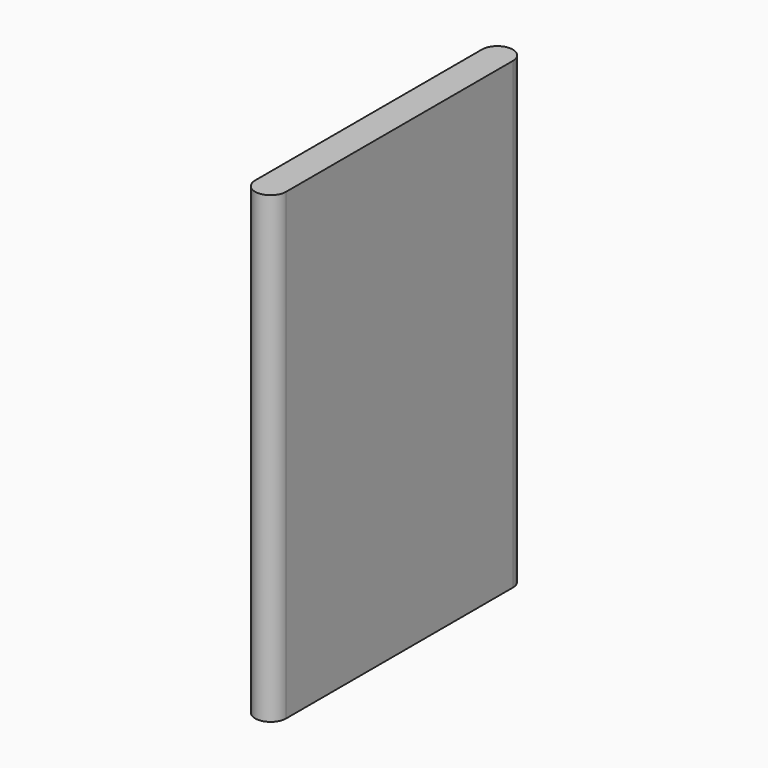
from build123d import *

# Parameters (mm, degrees)
F1_DEPTH     = 90
F2_TEXT_SIZE = 16.9558881971
F3_DEPTH     = 0.5


# Not quite as in the source:
# - Text() gives the source's letters only with a copy of the font that has no kerning and outlines rounded to 1/6400 em; it was checked with that copy


with BuildPart() as f1:
    # F0 (on Top) → F1 (new body)
    with BuildSketch(Plane.XY):
        with BuildLine():
            ThreePointArc((3, 27.5), (0, 30.5), (-3, 27.5))
            Line((-3, 27.5), (-3, -27.5))
            ThreePointArc((-3, -27.5), (0, -30.5), (3, -27.5))
            Line((3, -27.5), (3, 27.5))
        make_face()
    extrude(amount=F1_DEPTH)

    # F2 (on face) → F3 (cut)
    with BuildSketch(Plane(origin=(-3, 0, 0), x_dir=(0, -1, 0), z_dir=(-1, 0, 0))):
        with Locations(Location((-7.2917604981, 22.6235262949), (0, 0, 90))):
            Text('Merry', F2_TEXT_SIZE, font='Open Sans', text_align=(TextAlign.LEFT, TextAlign.BOTTOM))
        with Locations(Location((15.76824745, 5), (0, 0, 90))):
            Text('Christmas', F2_TEXT_SIZE, font='Open Sans', text_align=(TextAlign.LEFT, TextAlign.BOTTOM))
    extrude(amount=-F3_DEPTH, mode=Mode.SUBTRACT)


solid = f1.part
